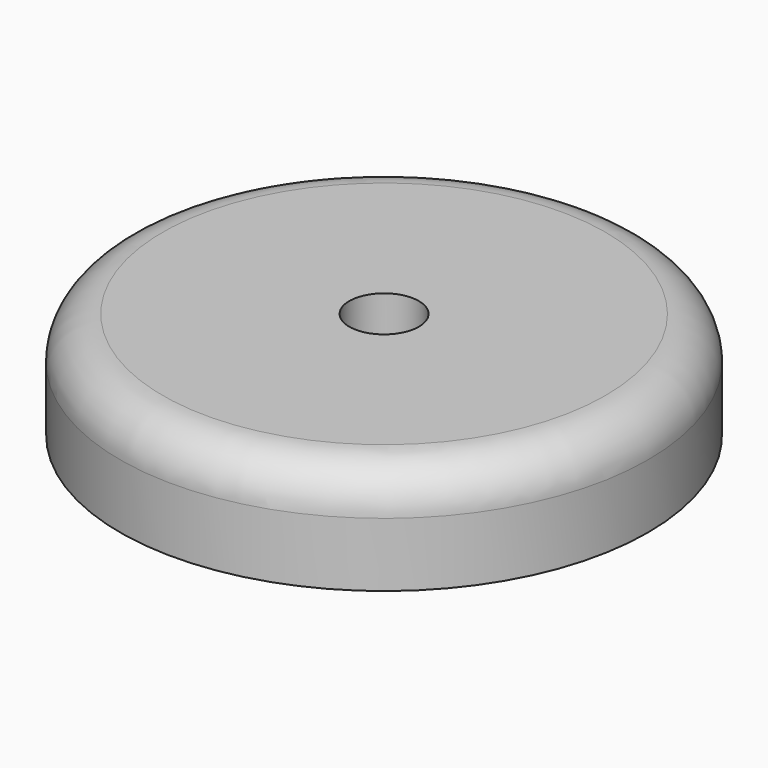
from build123d import *

# Parameters (mm, degrees)
F0_R     = 62.8660766499
F0_R_2   = 8.2840068325
F1_DEPTH = 25.4
F3_R     = 10.16


# Not quite as in the source:
# - the program builds the solid bodies; features that only make, move or delete a surface that nothing else refers to are left out


with BuildPart() as f1:
    # F0 (on Top) → F1 (new body)
    with BuildSketch(Plane.XY):
        Circle(F0_R)
        Circle(F0_R_2, mode=Mode.SUBTRACT)
    extrude(amount=F1_DEPTH)

    # F3
    f3_edges = [f1.edges().sort_by_distance(p)[0] for p in [
        (-62.866077, 0, 25.4),
    ]]
    fillet(f3_edges, radius=F3_R)


solid = f1.part
